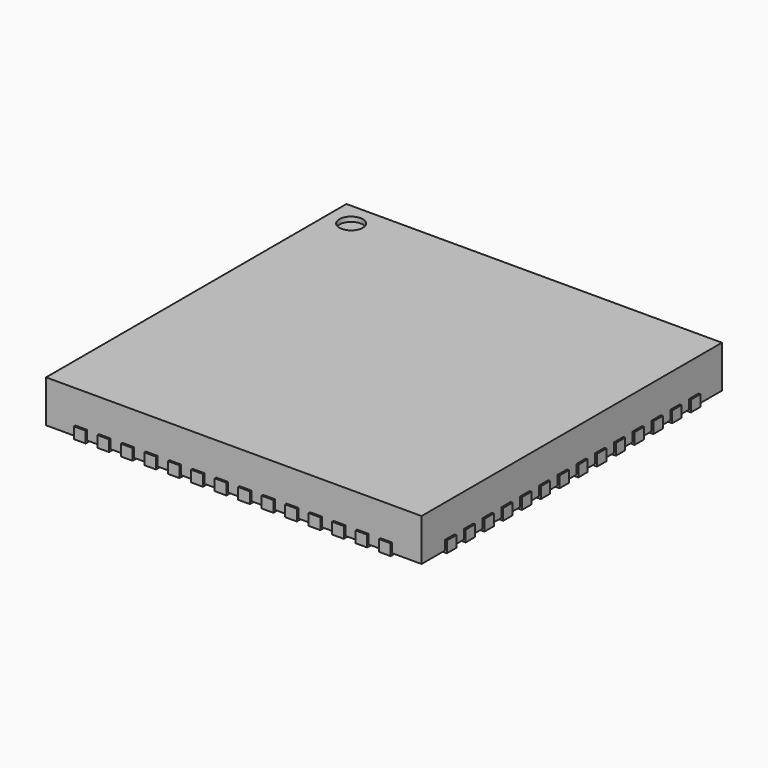
from build123d import *

# Parameters (mm, degrees)
F0_W      = 8
F0_H      = 8
F1_DEPTH  = 0.9
F2_R      = 0.25
F3_DEPTH  = 0.1
F6_W      = 7.2
F6_H      = 7.2
F7_DEPTH  = 0.1
F5_W      = 0.44
F5_H      = 0.25
F5_W_2    = 0.25
F5_H_2    = 0.44
F8_DEPTH  = 0.24
F10_DEPTH = 0.04


with BuildPart() as f1:
    # F0 (on Top) → F1 (new body)
    with BuildSketch(Plane.XY):
        Rectangle(F0_W, F0_H)
    extrude(amount=F1_DEPTH)

    # F2 (on face) → F3 (cut)
    with BuildSketch(Plane.XY.offset(0.9)):
        with Locations((-3.5, 3.5)):
            Circle(F2_R)
    extrude(amount=-F3_DEPTH, mode=Mode.SUBTRACT)


with BuildPart() as f7:
    # F6 (on offset) → F7 (new body)
    with BuildSketch(Plane.XY.offset(0.2)):
        Rectangle(F6_W, F6_H)
    extrude(amount=-F7_DEPTH)

    # F5 (on offset) → F8 (join)
    with BuildSketch(Plane.XY.offset(0.2)):
        with Locations((3.82, -2.75)):
            Rectangle(F5_W, F5_H)
        with Locations((3.82, -2.25)):
            Rectangle(F5_W, F5_H)
        with Locations((3.82, -1.75)):
            Rectangle(F5_W, F5_H)
        with Locations((3.82, -1.25)):
            Rectangle(F5_W, F5_H)
        with Locations((3.82, -0.75)):
            Rectangle(F5_W, F5_H)
        with Locations((3.82, -0.25)):
            Rectangle(F5_W, F5_H)
        Polygon((4.04, -3.125), (3.6, -3.125), (3.6, -3.325), (3.65, -3.375), (4.04, -3.375), align=None)
        Polygon((3.125, -4.04), (3.375, -4.04), (3.375, -3.65), (3.325, -3.6), (3.125, -3.6), align=None)
        with Locations((0.25, -3.82)):
            Rectangle(F5_W_2, F5_H_2)
        with Locations((1.75, -3.82)):
            Rectangle(F5_W_2, F5_H_2)
        with Locations((2.25, -3.82)):
            Rectangle(F5_W_2, F5_H_2)
        with Locations((2.75, -3.82)):
            Rectangle(F5_W_2, F5_H_2)
        with Locations((1.25, -3.82)):
            Rectangle(F5_W_2, F5_H_2)
        with Locations((0.75, -3.82)):
            Rectangle(F5_W_2, F5_H_2)
        Polygon((-3.125, -3.6), (-3.325, -3.6), (-3.375, -3.65), (-3.375, -4.04), (-3.125, -4.04), align=None)
        Polygon((-4.04, -3.375), (-3.65, -3.375), (-3.6, -3.325), (-3.6, -3.125), (-4.04, -3.125), align=None)
        with Locations((-3.82, -2.25)):
            Rectangle(F5_W, F5_H)
        with Locations((-3.82, -1.75)):
            Rectangle(F5_W, F5_H)
        with Locations((-0.75, -3.82)):
            Rectangle(F5_W_2, F5_H_2)
        with Locations((-0.25, -3.82)):
            Rectangle(F5_W_2, F5_H_2)
        with Locations((-3.82, -0.25)):
            Rectangle(F5_W, F5_H)
        with Locations((-1.75, -3.82)):
            Rectangle(F5_W_2, F5_H_2)
        with Locations((-2.75, -3.82)):
            Rectangle(F5_W_2, F5_H_2)
        with Locations((-3.82, -2.75)):
            Rectangle(F5_W, F5_H)
        with Locations((-3.82, -1.25)):
            Rectangle(F5_W, F5_H)
        with Locations((-2.25, -3.82)):
            Rectangle(F5_W_2, F5_H_2)
        with Locations((-1.25, -3.82)):
            Rectangle(F5_W_2, F5_H_2)
        with Locations((-3.82, -0.75)):
            Rectangle(F5_W, F5_H)
        Polygon((3.125, 3.6), (3.325, 3.6), (3.375, 3.65), (3.375, 4.04), (3.125, 4.04), align=None)
        Polygon((-3.125, 3.6), (-3.125, 4.04), (-3.375, 4.04), (-3.375, 3.65), (-3.325, 3.6), align=None)
        Polygon((4.04, 3.375), (3.65, 3.375), (3.6, 3.325), (3.6, 3.125), (4.04, 3.125), align=None)
        with Locations((-3.82, 0.25)):
            Rectangle(F5_W, F5_H)
        with Locations((0.75, 3.82)):
            Rectangle(F5_W_2, F5_H_2)
        with Locations((-3.82, 0.75)):
            Rectangle(F5_W, F5_H)
        with Locations((-3.82, 2.25)):
            Rectangle(F5_W, F5_H)
        with Locations((-3.82, 1.25)):
            Rectangle(F5_W, F5_H)
        with Locations((1.75, 3.82)):
            Rectangle(F5_W_2, F5_H_2)
        with Locations((-0.25, 3.82)):
            Rectangle(F5_W_2, F5_H_2)
        with Locations((-1.25, 3.82)):
            Rectangle(F5_W_2, F5_H_2)
        with Locations((-3.82, 2.75)):
            Rectangle(F5_W, F5_H)
        with Locations((-0.75, 3.82)):
            Rectangle(F5_W_2, F5_H_2)
        with Locations((-1.75, 3.82)):
            Rectangle(F5_W_2, F5_H_2)
        with Locations((-3.82, 1.75)):
            Rectangle(F5_W, F5_H)
        with Locations((1.25, 3.82)):
            Rectangle(F5_W_2, F5_H_2)
        Polygon((-3.6, 3.325), (-3.65, 3.375), (-4.04, 3.375), (-4.04, 3.125), (-3.6, 3.125), align=None)
        with Locations((2.25, 3.82)):
            Rectangle(F5_W_2, F5_H_2)
        with Locations((-2.75, 3.82)):
            Rectangle(F5_W_2, F5_H_2)
        with Locations((0.25, 3.82)):
            Rectangle(F5_W_2, F5_H_2)
        with Locations((3.82, 0.75)):
            Rectangle(F5_W, F5_H)
        with Locations((-2.25, 3.82)):
            Rectangle(F5_W_2, F5_H_2)
        with Locations((3.82, 0.25)):
            Rectangle(F5_W, F5_H)
        with Locations((2.75, 3.82)):
            Rectangle(F5_W_2, F5_H_2)
        with Locations((3.82, 1.75)):
            Rectangle(F5_W, F5_H)
        with Locations((3.82, 2.25)):
            Rectangle(F5_W, F5_H)
        with Locations((3.82, 1.25)):
            Rectangle(F5_W, F5_H)
        with Locations((3.82, 2.75)):
            Rectangle(F5_W, F5_H)
    extrude(amount=-F8_DEPTH)


with BuildPart() as f10:
    # F9 (on Top) → F10 (new body)
    with BuildSketch(Plane.XY):
        Polygon((-3, -3), (3, -3), (3, 3), (-2.65, 3), (-3, 2.65), align=None)
    extrude(amount=-F10_DEPTH)


solid = Compound([f1.part, f7.part, f10.part])
